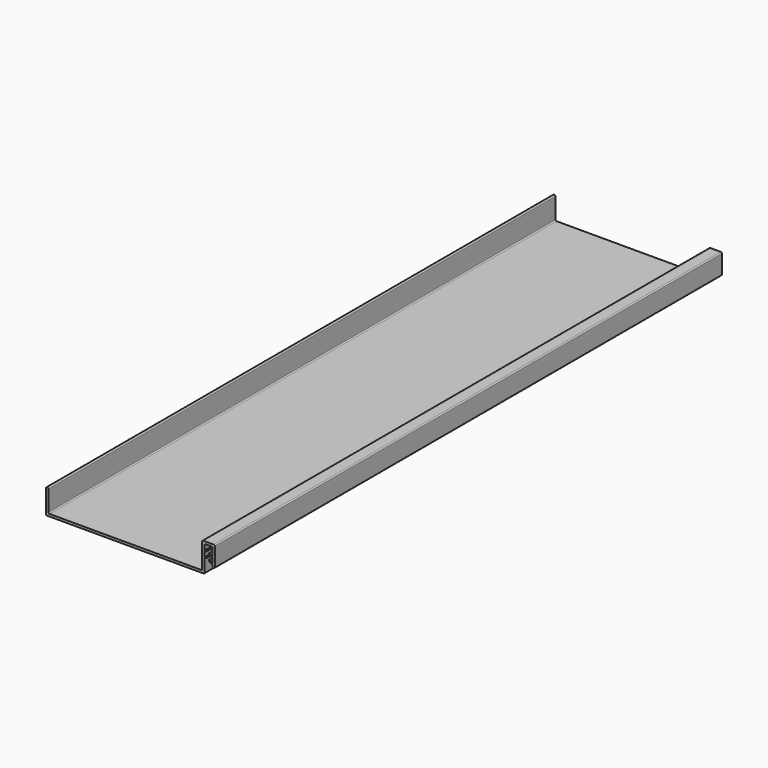
from build123d import *

# Parameters (mm, degrees)
F1_DEPTH = 609.6
F2_SCALE = 0.5


# Not quite as in the source:
# - ends of sketch curves that miss each other by under 0.0002 mm in the source are joined


with BuildPart() as f1:
    # F0 (on Front) → F1 (new body)
    with BuildSketch(Plane.XZ):
        with BuildLine():
            Line((-475.3549548, -393.1385076), (-475.3549548, -380.6970975265))
            ThreePointArc((-475.3549548, -380.6970975265), (-475.3563898659, -380.697073864), (-475.3578249233, -380.6970496949))
            ThreePointArc((-475.3578249233, -380.6970496949), (-475.5014064418, -380.6125311151), (-475.5028342338, -380.4459240484))
            ThreePointArc((-475.5028342338, -380.4459240484), (-475.4310666689, -380.3217397475), (-475.3549548, -380.2001693517))
            Line((-475.3549548, -380.2001693517), (-475.3549548, -374.9508555265))
            ThreePointArc((-475.3549548, -374.9508555265), (-475.356390082, -374.9508318604), (-475.3578253555, -374.9508076876))
            ThreePointArc((-475.3578253555, -374.9508076876), (-475.5014064418, -374.8662637151), (-475.5028342338, -374.6996566484))
            ThreePointArc((-475.5028342338, -374.6996566484), (-475.4310609426, -374.5754882319), (-475.3549548, -374.4539273517))
            Line((-475.3549548, -374.4539273517), (-475.3549548, -369.7705076))
            ThreePointArc((-475.3549548, -369.7705076), (-475.0573752897, -369.0520871103), (-474.3389548, -368.7545076))
            Line((-474.3389548, -368.7545076), (-468.7509548, -368.7545076))
            ThreePointArc((-468.7509548, -368.7545076), (-468.0325343103, -369.0520871103), (-467.7349548, -369.7705076))
            Line((-467.7349548, -369.7705076), (-467.7349548, -377.4055678497))
            ThreePointArc((-467.7349548, -377.4055678497), (-467.6588433745, -377.5271215868), (-467.5870659133, -377.6512838039))
            ThreePointArc((-467.5870659133, -377.6512838039), (-467.5884969176, -377.8178853065), (-467.7320596244, -377.9024198158))
            ThreePointArc((-467.7320596244, -377.9024198158), (-467.7335070711, -377.9024602361), (-467.7349548, -377.9024841911))
            Line((-467.7349548, -377.9024841911), (-467.7349548, -382.9365702497))
            ThreePointArc((-467.7349548, -382.9365702497), (-467.6588433745, -383.0581239868), (-467.5870659133, -383.1822862039))
            ThreePointArc((-467.5870659133, -383.1822862039), (-467.5884968089, -383.3488875182), (-467.7320591896, -383.4334222084))
            ThreePointArc((-467.7320591896, -383.4334222084), (-467.7335068543, -383.4334626325), (-467.7349548, -383.4334865911))
            Line((-467.7349548, -383.4334865911), (-467.7349548, -385.2645076))
            ThreePointArc((-467.7349548, -385.2645076), (-467.4373752897, -385.9829280897), (-466.7189548, -386.2805076))
            Line((-466.7189548, -386.2805076), (-466.4649548, -386.2805076))
            ThreePointArc((-466.4649548, -386.2805076), (-465.7465343103, -385.9829280897), (-465.4489548, -385.2645076))
            Line((-465.4489548, -385.2645076), (-465.4489548, -367.4845076))
            ThreePointArc((-465.4489548, -367.4845076), (-465.7465343103, -366.7660871103), (-466.4649548, -366.4685076))
            Line((-466.4649548, -366.4685076), (-476.6249548, -366.4685076))
            ThreePointArc((-476.6249548, -366.4685076), (-477.3433752897, -366.7660871103), (-477.6409548, -367.4845076))
            Line((-477.6409548, -367.4845076), (-477.6409548, -390.8525076))
            ThreePointArc((-477.6409548, -390.8525076), (-477.9385343103, -391.5709280897), (-478.6569548, -391.8685076))
            Line((-478.6569548, -391.8685076), (-624.4529548, -391.8685076))
            ThreePointArc((-624.4529548, -391.8685076), (-625.1713752897, -391.5709280897), (-625.4689548, -390.8525076))
            Line((-625.4689548, -390.8525076), (-625.4689548, -371.0405076))
            ThreePointArc((-625.4689548, -371.0405076), (-625.7665343103, -370.3220871103), (-626.4849548, -370.0245076))
            Line((-626.4849548, -370.0245076), (-626.7389548, -370.0245076))
            ThreePointArc((-626.7389548, -370.0245076), (-627.4573752897, -370.3220871103), (-627.7549548, -371.0405076))
            Line((-627.7549548, -371.0405076), (-627.7549548, -393.1385076))
            ThreePointArc((-627.7549548, -393.1385076), (-627.4573752897, -393.8569280897), (-626.7389548, -394.1545076))
            Line((-626.7389548, -394.1545076), (-476.3709548, -394.1545076))
            ThreePointArc((-476.3709548, -394.1545076), (-475.6525343103, -393.8569280897), (-475.3549548, -393.1385076))
        make_face()
    extrude(amount=F1_DEPTH)


with BuildPart() as f1b:
    # F0 (on Front) → F1, piece 2 (new body)
    with BuildSketch(Plane.XZ):
        with BuildLine():
            Line((-475.3549548, -374.4539273517), (-475.3549548, -374.9508555265))
            ThreePointArc((-475.3549548, -374.9508555265), (-473.2540858532, -374.4057852487), (-471.7328988759, -372.8576437436))
            ThreePointArc((-471.7328988759, -372.8576437436), (-471.7343450388, -372.6910369501), (-471.8779233823, -372.6065181587))
            ThreePointArc((-471.8779233823, -372.6065181587), (-473.8549585951, -373.0813038086), (-475.3549548, -374.4539273517))
        make_face()
    extrude(amount=F1_DEPTH)


with BuildPart() as f1c:
    # F0 (on Front) → F1, piece 3 (new body)
    with BuildSketch(Plane.XZ):
        with BuildLine():
            Line((-467.7349548, -377.9024841911), (-467.7349548, -377.4055678497))
            ThreePointArc((-467.7349548, -377.4055678497), (-469.2350389344, -376.0330252213), (-471.2121130491, -375.5583636344))
            ThreePointArc((-471.2121130491, -375.5583636344), (-471.355694534, -375.6429030983), (-471.3571224338, -375.8095103516))
            ThreePointArc((-471.3571224338, -375.8095103516), (-469.835840158, -377.3575402656), (-467.7349548, -377.9024841911))
        make_face()
    extrude(amount=F1_DEPTH)


with BuildPart() as f1d:
    # F0 (on Front) → F1, piece 4 (new body)
    with BuildSketch(Plane.XZ):
        with BuildLine():
            ThreePointArc((-475.3549548, -380.6970975265), (-473.2540954687, -380.1520328055), (-471.7329096502, -378.6039051668))
            ThreePointArc((-471.7329096502, -378.6039051668), (-471.7343450388, -378.4373043501), (-471.8779233823, -378.3527855587))
            ThreePointArc((-471.8779233823, -378.3527855587), (-473.8549584042, -378.8275457072), (-475.3549548, -380.2001693517))
            Line((-475.3549548, -380.2001693517), (-475.3549548, -380.6970975265))
        make_face()
    extrude(amount=F1_DEPTH)


with BuildPart() as f1e:
    # F0 (on Front) → F1, piece 5 (new body)
    with BuildSketch(Plane.XZ):
        with BuildLine():
            Line((-467.7349548, -383.4334865911), (-467.7349548, -382.9365702497))
            ThreePointArc((-467.7349548, -382.9365702497), (-469.2350389344, -381.5640276213), (-471.2121130491, -381.0893660344))
            ThreePointArc((-471.2121130491, -381.0893660344), (-471.3557001943, -381.1738899017), (-471.3571116581, -381.3405067716))
            ThreePointArc((-471.3571116581, -381.3405067716), (-469.835840158, -382.8885426656), (-467.7349548, -383.4334865911))
        make_face()
    extrude(amount=F1_DEPTH)


with BuildPart() as f1d_1:
    # F2: moved
    add(f1d.part.scale(F2_SCALE))


with BuildPart() as f1_1:
    # F2: moved
    add(f1.part.scale(F2_SCALE))


with BuildPart() as f1b_1:
    # F2: moved
    add(f1b.part.scale(F2_SCALE))


with BuildPart() as f1e_1:
    # F2: moved
    add(f1e.part.scale(F2_SCALE))


with BuildPart() as f1c_1:
    # F2: moved
    add(f1c.part.scale(F2_SCALE))


solid = Compound([f1d_1.part, f1_1.part, f1b_1.part, f1e_1.part, f1c_1.part])
